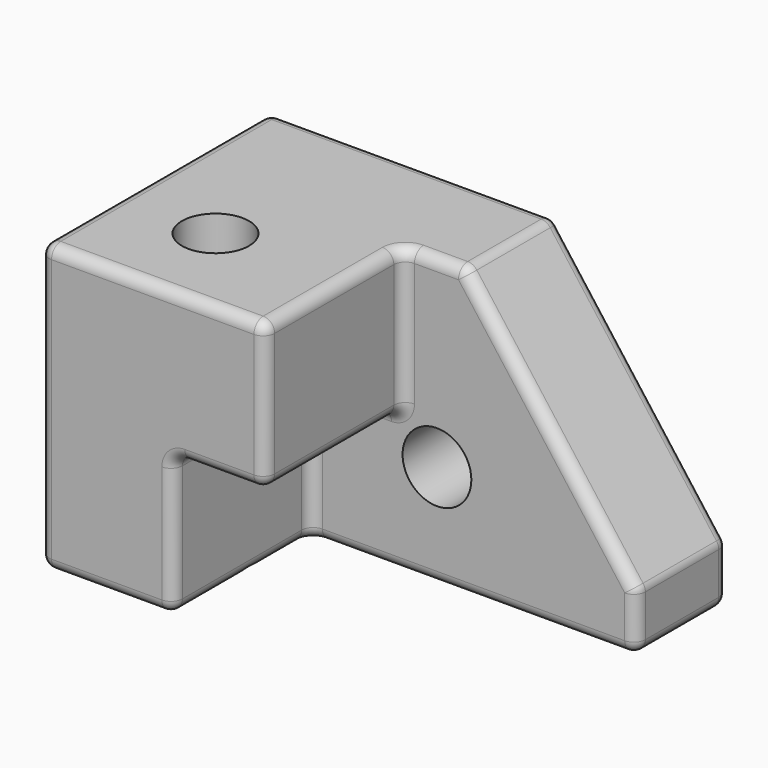
from build123d import *

# Parameters (mm, degrees)
F0_W     = 203.2
F0_H     = 127
F1_DEPTH = 127
F3_DEPTH = 76.2
F4_SIZE2 = 101.6
F4_SIZE  = 76.2
F5_R     = 5.08
F6_R     = 15.24
F7_DEPTH = 50.8
F8_R     = 14.8914565461
F9_DEPTH = 127


with BuildPart() as f1:
    # F0 (on Front) → F1 (new body)
    with BuildSketch(Plane.XZ):
        with Locations((1.736553802, 1.4607831836)):
            Rectangle(F0_W, F0_H)
    extrude(amount=F1_DEPTH)

    # F2 (on face) → F3 (cut)
    with BuildSketch(Plane.XZ.offset(127)):
        Polygon((0, 64.9607831836), (0, 0), (-40.8341363072, 0), (-40.8341363072, -62.0392168164), (103.336553802, -62.0392168164), (103.336553802, 64.9607831836), align=None)
    extrude(amount=-F3_DEPTH, mode=Mode.SUBTRACT)

    # F4
    f4_edges = [f1.edges().sort_by_distance(p)[0] for p in [
        (103.336554, -25.4, 64.960783),
    ]]
    f4_side = f1.faces().sort_by_distance((-20.189124, -52.346525, 64.960783))[0]
    chamfer(f4_edges, length=F4_SIZE, length2=F4_SIZE2, reference=f4_side)

    # F5
    f5_edges = [f1.edges().sort_by_distance(p)[0] for p in [
        (-99.863446, -63.5, 64.960783),
        (-49.931723, -127, 64.960783),
        (0, -88.9, 64.960783),
        (27.136554, -25.4, 64.960783),
        (13.568277, -50.8, 64.960783),
        (65.236554, -50.8, 14.160783),
        (0, -50.8, 32.480392),
        (0, -127, 32.480392),
        (31.251209, -50.8, -62.039217),
        (103.336554, -50.8, -49.339217),
        (103.336554, -25.4, -36.639217),
        (103.336554, -25.4, -62.039217),
        (103.336554, 0, -49.339217),
        (65.236554, 0, 14.160783),
        (-20.417068, -127, 0),
        (-40.834136, -127, -31.019608),
        (-40.834136, -88.9, -62.039217),
        (-40.834136, -50.8, -31.019608),
        (0, -88.9, 0),
        (-40.834136, -88.9, 0),
        (-99.863446, -63.5, -62.039217),
        (-70.348791, -127, -62.039217),
        (1.736554, 0, -62.039217),
        (-99.863446, -127, 1.460783),
        (-99.863446, 0, 1.460783),
        (-36.363446, 0, 64.960783),
        (-20.417068, -50.8, 0),
    ]]
    fillet(f5_edges, radius=F5_R)

    # F6 (on face) → F7 (cut, through all)
    with BuildSketch(Plane.XZ.offset(50.8)):
        with Locations((15.0458636928, -16.3192168164)):
            Circle(F6_R)
    extrude(amount=-F7_DEPTH, mode=Mode.SUBTRACT)

    # F8 (on face) → F9 (cut, through all)
    with BuildSketch(Plane.XY.offset(64.9607831836)):
        with Locations((-56.683446198, -83.82)):
            Circle(F8_R)
    extrude(amount=-F9_DEPTH, mode=Mode.SUBTRACT)


solid = f1.part
